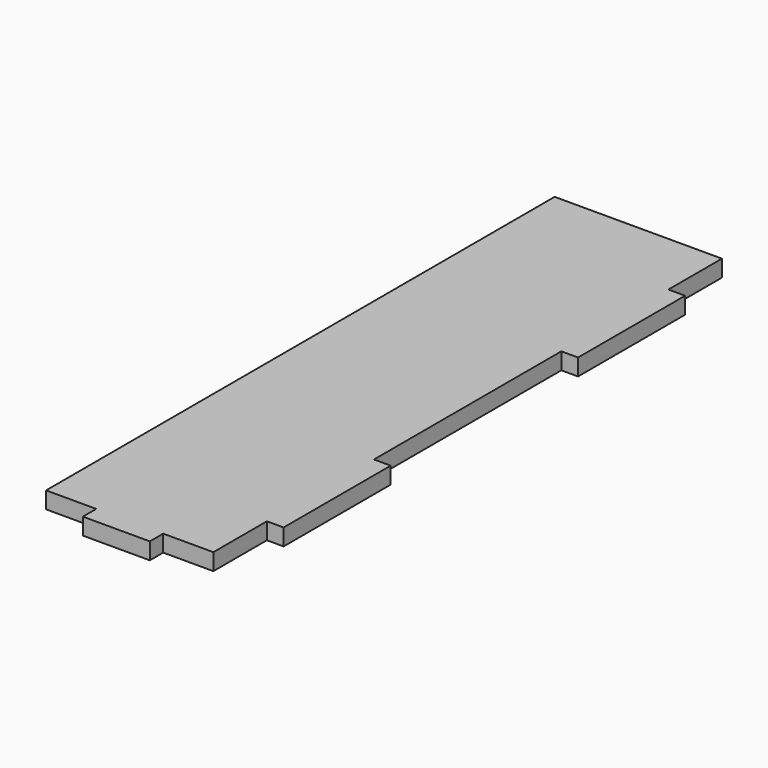
from build123d import *

# Parameters (mm, degrees)
F0_W     = 63.5
F0_H     = 241.3
F1_DEPTH = 6.35
F2_W     = 6.35
F2_H     = 50.8
F3_DEPTH = 6.35
F4_W     = 25.4
F4_H     = 6.35
F5_DEPTH = 6.35


# Not quite as in the source:
# - a pattern or mirror of a feature is missing from the dataset's text; its kind, count and spacing are read off the source's solid


with BuildPart() as f1:
    # F0 (on Top) → F1 (new body)
    with BuildSketch(Plane.XY):
        with Locations((31.75, 0)):
            Rectangle(F0_W, F0_H)
    extrude(amount=F1_DEPTH)

    # F2 (on face) → F3 (join)
    with BuildSketch(Plane.XY.offset(6.35)):
        with Locations((66.675, 69.85)):
            Rectangle(F2_W, F2_H)
    f3 = extrude(amount=-F3_DEPTH)

    # F3_copies: F3 across plane
    add(f3.mirror(Plane(origin=(0, 0, 0), x_dir=(0, 0, -1), z_dir=(0, -1, 0))))

    # F4 (on face) → F5 (join)
    with BuildSketch(Plane.XY.offset(6.35)):
        with Locations((31.75, -123.825)):
            Rectangle(F4_W, F4_H)
    extrude(amount=-F5_DEPTH)


solid = f1.part
